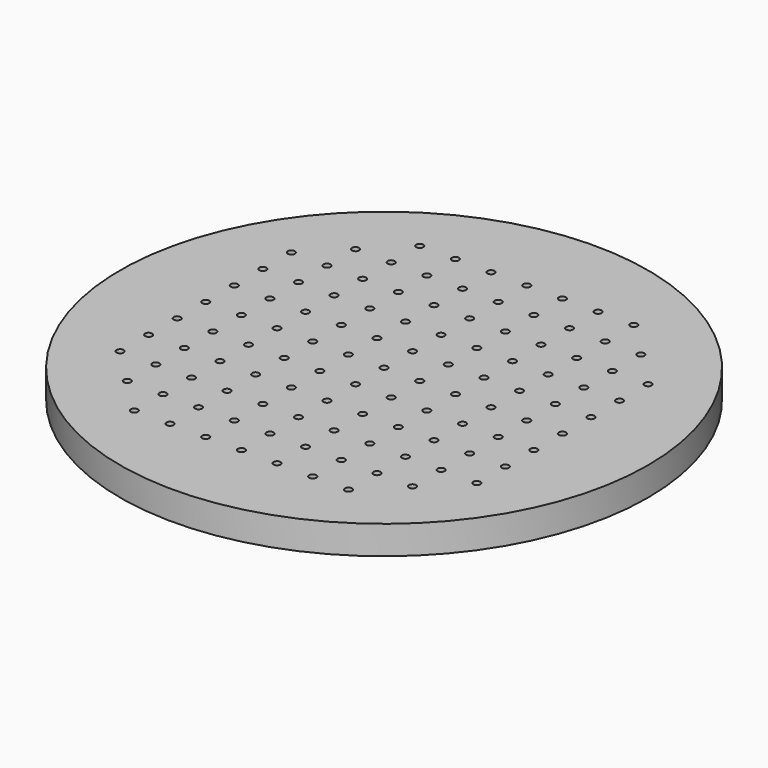
from build123d import *

# Parameters (mm, degrees)
F0_R     = 185
F1_DEPTH = 20
F4_R     = 2.5
F5_DEPTH = 5


# Not quite as in the source:
# - the program builds the solid bodies; features that only make, move or delete a surface that nothing else refers to are left out


with BuildPart() as f1:
    # F0 (on Top) → F1 (new body)
    with BuildSketch(Plane.XY):
        Circle(F0_R)
    extrude(amount=F1_DEPTH)

    # F4 (on face) → F5 (cut)
    with BuildSketch(Plane.XY.offset(20)):
        Circle(F4_R)
        with Locations((0, 25)):
            Circle(F4_R)
        with Locations((0, 50)):
            Circle(F4_R)
        with Locations((0, 75)):
            Circle(F4_R)
        with Locations((0, 100)):
            Circle(F4_R)
        with Locations((0, 125)):
            Circle(F4_R)
        with Locations((25, 0)):
            Circle(F4_R)
        with Locations((25, 25)):
            Circle(F4_R)
        with Locations((25, 50)):
            Circle(F4_R)
        with Locations((25, 75)):
            Circle(F4_R)
        with Locations((25, 100)):
            Circle(F4_R)
        with Locations((25, 125)):
            Circle(F4_R)
        with Locations((50, 0)):
            Circle(F4_R)
        with Locations((50, 25)):
            Circle(F4_R)
        with Locations((50, 50)):
            Circle(F4_R)
        with Locations((50, 75)):
            Circle(F4_R)
        with Locations((50, 100)):
            Circle(F4_R)
        with Locations((50, 125)):
            Circle(F4_R)
        with Locations((75, 0)):
            Circle(F4_R)
        with Locations((75, 25)):
            Circle(F4_R)
        with Locations((75, 50)):
            Circle(F4_R)
        with Locations((75, 75)):
            Circle(F4_R)
        with Locations((75, 100)):
            Circle(F4_R)
        with Locations((75, 125)):
            Circle(F4_R)
        with Locations((100, 0)):
            Circle(F4_R)
        with Locations((100, 25)):
            Circle(F4_R)
        with Locations((100, 50)):
            Circle(F4_R)
        with Locations((100, 75)):
            Circle(F4_R)
        with Locations((100, 100)):
            Circle(F4_R)
        with Locations((125, 0)):
            Circle(F4_R)
        with Locations((125, 25)):
            Circle(F4_R)
        with Locations((125, 50)):
            Circle(F4_R)
        with Locations((125, 75)):
            Circle(F4_R)
        with Locations((75, -25)):
            Circle(F4_R)
        with Locations((100, -50)):
            Circle(F4_R)
        with Locations((0, -100)):
            Circle(F4_R)
        with Locations((100, -100)):
            Circle(F4_R)
        with Locations((75, -100)):
            Circle(F4_R)
        with Locations((125, -50)):
            Circle(F4_R)
        with Locations((75, -125)):
            Circle(F4_R)
        with Locations((25, -50)):
            Circle(F4_R)
        with Locations((0, -75)):
            Circle(F4_R)
        with Locations((100, -75)):
            Circle(F4_R)
        with Locations((100, -25)):
            Circle(F4_R)
        with Locations((50, -125)):
            Circle(F4_R)
        with Locations((125, -25)):
            Circle(F4_R)
        with Locations((50, -75)):
            Circle(F4_R)
        with Locations((25, -25)):
            Circle(F4_R)
        with Locations((75, -75)):
            Circle(F4_R)
        with Locations((75, -50)):
            Circle(F4_R)
        with Locations((125, -75)):
            Circle(F4_R)
        with Locations((0, -125)):
            Circle(F4_R)
        with Locations((25, -75)):
            Circle(F4_R)
        with Locations((50, -100)):
            Circle(F4_R)
        with Locations((25, -125)):
            Circle(F4_R)
        with Locations((0, -50)):
            Circle(F4_R)
        with Locations((25, -100)):
            Circle(F4_R)
        with Locations((50, -25)):
            Circle(F4_R)
        with Locations((50, -50)):
            Circle(F4_R)
        with Locations((0, -25)):
            Circle(F4_R)
        with Locations((-25, -75)):
            Circle(F4_R)
        with Locations((-50, -100)):
            Circle(F4_R)
        with Locations((-100, 0)):
            Circle(F4_R)
        with Locations((-100, -100)):
            Circle(F4_R)
        with Locations((-100, -75)):
            Circle(F4_R)
        with Locations((-50, -125)):
            Circle(F4_R)
        with Locations((-125, -75)):
            Circle(F4_R)
        with Locations((-50, -25)):
            Circle(F4_R)
        with Locations((-75, 0)):
            Circle(F4_R)
        with Locations((-75, -100)):
            Circle(F4_R)
        with Locations((-25, -100)):
            Circle(F4_R)
        with Locations((-125, -50)):
            Circle(F4_R)
        with Locations((-25, -125)):
            Circle(F4_R)
        with Locations((-75, -50)):
            Circle(F4_R)
        with Locations((-25, -25)):
            Circle(F4_R)
        with Locations((-75, -75)):
            Circle(F4_R)
        with Locations((-50, -75)):
            Circle(F4_R)
        with Locations((-75, -125)):
            Circle(F4_R)
        with Locations((-125, 0)):
            Circle(F4_R)
        with Locations((-75, -25)):
            Circle(F4_R)
        with Locations((-100, -50)):
            Circle(F4_R)
        with Locations((-125, -25)):
            Circle(F4_R)
        with Locations((-50, 0)):
            Circle(F4_R)
        with Locations((-100, -25)):
            Circle(F4_R)
        with Locations((-25, -50)):
            Circle(F4_R)
        with Locations((-50, -50)):
            Circle(F4_R)
        with Locations((-25, 0)):
            Circle(F4_R)
        with Locations((-75, 25)):
            Circle(F4_R)
        with Locations((-100, 50)):
            Circle(F4_R)
        with Locations((-100, 100)):
            Circle(F4_R)
        with Locations((-75, 100)):
            Circle(F4_R)
        with Locations((-125, 50)):
            Circle(F4_R)
        with Locations((-75, 125)):
            Circle(F4_R)
        with Locations((-25, 50)):
            Circle(F4_R)
        with Locations((-100, 75)):
            Circle(F4_R)
        with Locations((-100, 25)):
            Circle(F4_R)
        with Locations((-50, 125)):
            Circle(F4_R)
        with Locations((-125, 25)):
            Circle(F4_R)
        with Locations((-50, 75)):
            Circle(F4_R)
        with Locations((-25, 25)):
            Circle(F4_R)
        with Locations((-75, 75)):
            Circle(F4_R)
        with Locations((-75, 50)):
            Circle(F4_R)
        with Locations((-125, 75)):
            Circle(F4_R)
        with Locations((-25, 75)):
            Circle(F4_R)
        with Locations((-50, 100)):
            Circle(F4_R)
        with Locations((-25, 125)):
            Circle(F4_R)
        with Locations((-25, 100)):
            Circle(F4_R)
        with Locations((-50, 25)):
            Circle(F4_R)
        with Locations((-50, 50)):
            Circle(F4_R)
    extrude(amount=-F5_DEPTH, mode=Mode.SUBTRACT)


solid = f1.part
